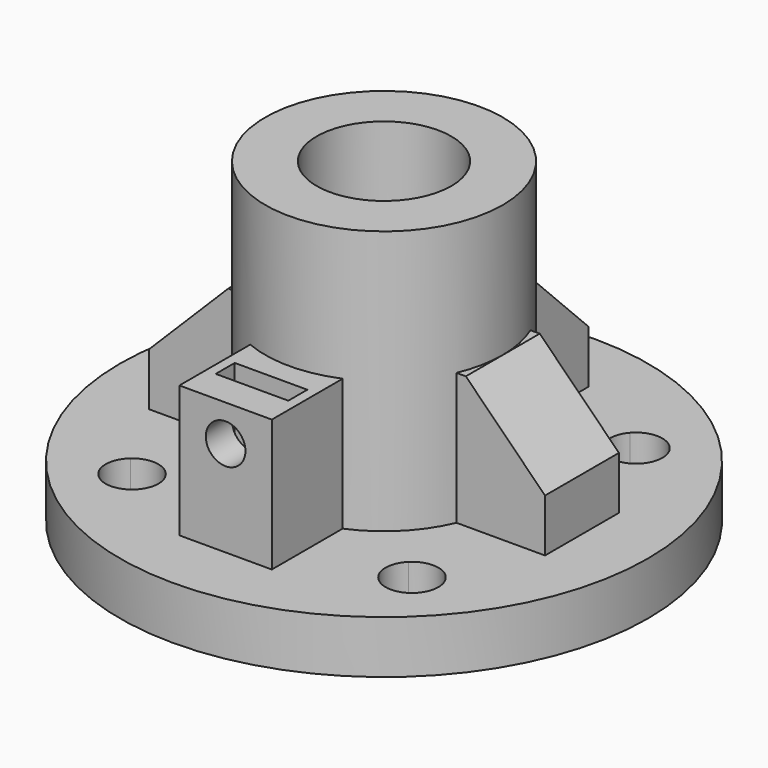
from build123d import *

# Parameters (mm, degrees)
F0_R      = 20
F1_DEPTH  = 4
F2_R      = 9
F2_R_2    = 5.1
F3_DEPTH  = 20
F5_DEPTH  = 10
F6_W      = 5.5
F6_H      = 1.8
F7_DEPTH  = 5.5
F8_R      = 1.5
F9_DEPTH  = 11
F10_SIZE  = 5.99999
F12_DEPTH = 25


# Not quite as in the source:
# - a fillet or chamfer is up to 0.001 mm smaller than in the source, because OpenCascade refuses the exact size


with BuildPart() as f1:
    # F0 (on Top) → F1 (new body)
    with BuildSketch(Plane.XY):
        Circle(F0_R)
    extrude(amount=F1_DEPTH)

    # F2 (on face) → F3 (join)
    with BuildSketch(Plane.XY.offset(4)):
        Circle(F2_R)
        Circle(F2_R_2, mode=Mode.SUBTRACT)
    extrude(amount=F3_DEPTH)

    # F4 (on face) → F5 (join)
    with BuildSketch(Plane.XY.offset(4)):
        with BuildLine():
            Line((-3.5, 15), (-3.5, 8.2915619759))
            ThreePointArc((-3.5, 8.2915619759), (0, 9), (3.5, 8.2915619759))
            Line((3.5, 8.2915619759), (3.5, 15))
            Line((3.5, 15), (-3.5, 15))
        make_face()
        with BuildLine():
            Line((15, 3.5), (8.2915619759, 3.5))
            ThreePointArc((8.2915619759, 3.5), (8.8211126788, 1.785489039), (9, 0))
            ThreePointArc((9, 0), (8.8211126788, -1.785489039), (8.2915619759, -3.5))
            Line((8.2915619759, -3.5), (15, -3.5))
            Line((15, -3.5), (15, 3.5))
        make_face()
        with BuildLine():
            Line((-8.2915619759, 3.5), (-15, 3.5))
            Line((-15, 3.5), (-15, -3.5))
            Line((-15, -3.5), (-8.2915619759, -3.5))
            ThreePointArc((-8.2915619759, -3.5), (-9, 0), (-8.2915619759, 3.5))
        make_face()
        with BuildLine():
            ThreePointArc((3.5, -8.2915619759), (0, -9), (-3.5, -8.2915619759))
            Line((-3.5, -8.2915619759), (-3.5, -15))
            Line((-3.5, -15), (3.5, -15))
            Line((3.5, -15), (3.5, -8.2915619759))
        make_face()
    extrude(amount=F5_DEPTH)

    # F6 (on face) → F7 (cut)
    with BuildSketch(Plane.XY.offset(14)):
        with Locations((0, -11.6)):
            Rectangle(F6_W, F6_H)
    extrude(amount=-F7_DEPTH, mode=Mode.SUBTRACT)

    # F8 (on face) → F9 (cut)
    with BuildSketch(Plane.XZ.offset(15)):
        with Locations((0, 11.25)):
            Circle(F8_R)
    extrude(amount=-F9_DEPTH, mode=Mode.SUBTRACT)

    # F10 (size 6 in the source; OpenCascade refuses exactly that, so slightly less here)
    f10_edges = [f1.edges().sort_by_distance(p)[0] for p in [
        (15, 0, 14),
        (0, 15, 14),
        (-15, 0, 14),
    ]]
    chamfer(f10_edges, length=F10_SIZE)

    # F11 (on face) → F12 (cut)
    with BuildSketch(Plane(origin=(0, 0, 0), x_dir=(1, 0, 0), z_dir=(0, 0, -1))):
        with BuildLine():
            ThreePointArc((-10.6066017178, 10.6066017178), (-9.8758984631, 11.2901120254), (-9.1012534477, 11.9233881795))
            ThreePointArc((-9.1012534477, 11.9233881795), (-12.0208152802, 12.0208152802), (-11.9233881795, 9.1012534477))
            ThreePointArc((-11.9233881795, 9.1012534477), (-11.2901120254, 9.8758984631), (-10.6066017178, 10.6066017178))
        make_face()
        with BuildLine():
            Line((-10.6066017178, 10.6066017178), (-9.1923881554, 9.1923881554))
            ThreePointArc((-9.1923881554, 9.1923881554), (-8.7588426528, 9.8412348531), (-8.6066017178, 10.6066017178))
            ThreePointArc((-8.6066017178, 10.6066017178), (-8.7343441847, 11.3099165335), (-9.1012534477, 11.9233881795))
            ThreePointArc((-9.1012534477, 11.9233881795), (-9.8758984631, 11.2901120254), (-10.6066017178, 10.6066017178))
        make_face()
        with BuildLine():
            ThreePointArc((-11.9233881795, 9.1012534477), (-10.5398979419, 8.6077143757), (-9.1923881554, 9.1923881554))
            Line((-9.1923881554, 9.1923881554), (-10.6066017178, 10.6066017178))
            ThreePointArc((-10.6066017178, 10.6066017178), (-11.2901120254, 9.8758984631), (-11.9233881795, 9.1012534477))
        make_face()
        with BuildLine():
            ThreePointArc((9.1923881554, 9.1923881554), (10.5398979419, 8.6077143757), (11.9233881795, 9.1012534477))
            ThreePointArc((11.9233881795, 9.1012534477), (11.2901120254, 9.8758984631), (10.6066017178, 10.6066017178))
            Line((10.6066017178, 10.6066017178), (9.1923881554, 9.1923881554))
        make_face()
        with BuildLine():
            ThreePointArc((10.6066017178, 10.6066017178), (11.2901120254, 9.8758984631), (11.9233881795, 9.1012534477))
            ThreePointArc((11.9233881795, 9.1012534477), (12.427806391, 9.7800343955), (12.6066017178, 10.6066017178))
            ThreePointArc((12.6066017178, 10.6066017178), (11.3099165335, 12.4788592508), (9.1012534477, 11.9233881795))
            ThreePointArc((9.1012534477, 11.9233881795), (9.8758984631, 11.2901120254), (10.6066017178, 10.6066017178))
        make_face()
        with BuildLine():
            Line((9.1923881554, 9.1923881554), (10.6066017178, 10.6066017178))
            ThreePointArc((10.6066017178, 10.6066017178), (9.8758984631, 11.2901120254), (9.1012534477, 11.9233881795))
            ThreePointArc((9.1012534477, 11.9233881795), (8.6077143757, 10.5398979419), (9.1923881554, 9.1923881554))
        make_face()
        with BuildLine():
            ThreePointArc((12.6066017178, -10.6066017178), (12.427806391, -9.7800343955), (11.9233881795, -9.1012534477))
            ThreePointArc((11.9233881795, -9.1012534477), (11.2901120254, -9.8758984631), (10.6066017178, -10.6066017178))
            ThreePointArc((10.6066017178, -10.6066017178), (9.8758984631, -11.2901120254), (9.1012534477, -11.9233881795))
            ThreePointArc((9.1012534477, -11.9233881795), (11.3099165335, -12.4788592508), (12.6066017178, -10.6066017178))
        make_face()
        with BuildLine():
            ThreePointArc((10.6066017178, -10.6066017178), (11.2901120254, -9.8758984631), (11.9233881795, -9.1012534477))
            ThreePointArc((11.9233881795, -9.1012534477), (10.5398979419, -8.6077143757), (9.1923881554, -9.1923881554))
            Line((9.1923881554, -9.1923881554), (10.6066017178, -10.6066017178))
        make_face()
        with BuildLine():
            ThreePointArc((9.1012534477, -11.9233881795), (9.8758984631, -11.2901120254), (10.6066017178, -10.6066017178))
            Line((10.6066017178, -10.6066017178), (9.1923881554, -9.1923881554))
            ThreePointArc((9.1923881554, -9.1923881554), (8.6077143757, -10.5398979419), (9.1012534477, -11.9233881795))
        make_face()
        with BuildLine():
            ThreePointArc((-11.9233881795, -9.1012534477), (-12.0208152802, -12.0208152802), (-9.1012534477, -11.9233881795))
            ThreePointArc((-9.1012534477, -11.9233881795), (-9.8758984631, -11.2901120254), (-10.6066017178, -10.6066017178))
            ThreePointArc((-10.6066017178, -10.6066017178), (-11.2901120254, -9.8758984631), (-11.9233881795, -9.1012534477))
        make_face()
        with BuildLine():
            ThreePointArc((-8.6066017178, -10.6066017178), (-8.7588426528, -9.8412348531), (-9.1923881554, -9.1923881554))
            Line((-9.1923881554, -9.1923881554), (-10.6066017178, -10.6066017178))
            ThreePointArc((-10.6066017178, -10.6066017178), (-9.8758984631, -11.2901120254), (-9.1012534477, -11.9233881795))
            ThreePointArc((-9.1012534477, -11.9233881795), (-8.7343441847, -11.3099165335), (-8.6066017178, -10.6066017178))
        make_face()
        with BuildLine():
            Line((-10.6066017178, -10.6066017178), (-9.1923881554, -9.1923881554))
            ThreePointArc((-9.1923881554, -9.1923881554), (-10.5398979419, -8.6077143757), (-11.9233881795, -9.1012534477))
            ThreePointArc((-11.9233881795, -9.1012534477), (-11.2901120254, -9.8758984631), (-10.6066017178, -10.6066017178))
        make_face()
    extrude(amount=-F12_DEPTH, mode=Mode.SUBTRACT)


solid = f1.part
